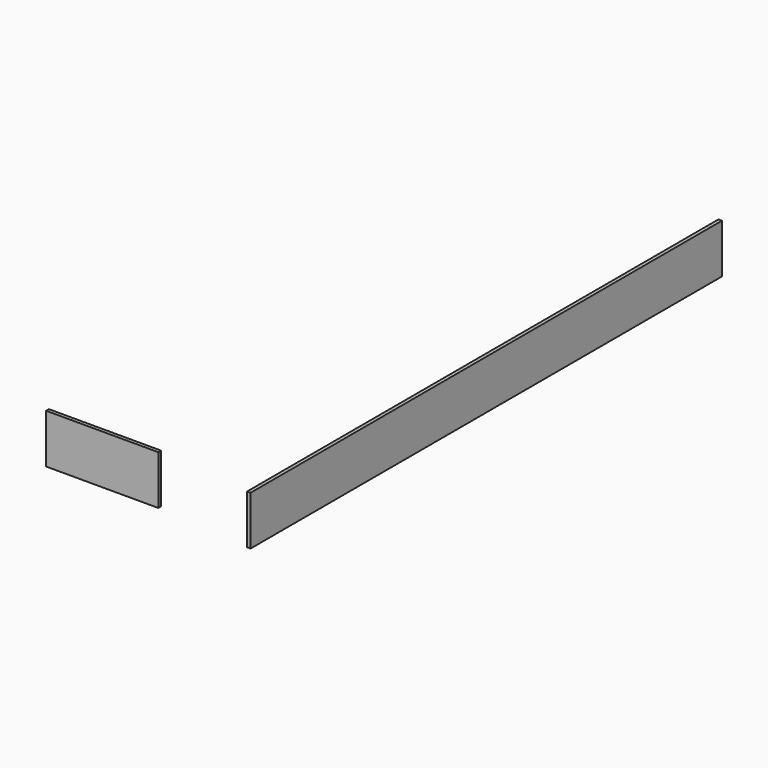
from build123d import *

# Parameters (mm, degrees)
F1_W     = 2133.6
F1_H     = 177.8
F2_DEPTH = 12.7
F3_W     = 406.4
F3_H     = 177.8
F4_DEPTH = 12.7


# Not quite as in the source:
# - a variable given as a bare number and used for a length is read in inches; the dataset says mm whatever the document's units were


with BuildPart() as f2:
    # F1 (on Right) → F2 (new body)
    with BuildSketch(Plane.YZ):
        with Locations((1002.147519815, 102.6993451208)):
            Rectangle(F1_W, F1_H)
    extrude(amount=F2_DEPTH)


with BuildPart() as f4:
    # F3 (on Front) → F4 (new body)
    with BuildSketch(Plane.XZ):
        with Locations((-565.90815534, 88.9)):
            Rectangle(F3_W, F3_H)
    extrude(amount=F4_DEPTH)


solid = Compound([f2.part, f4.part])
